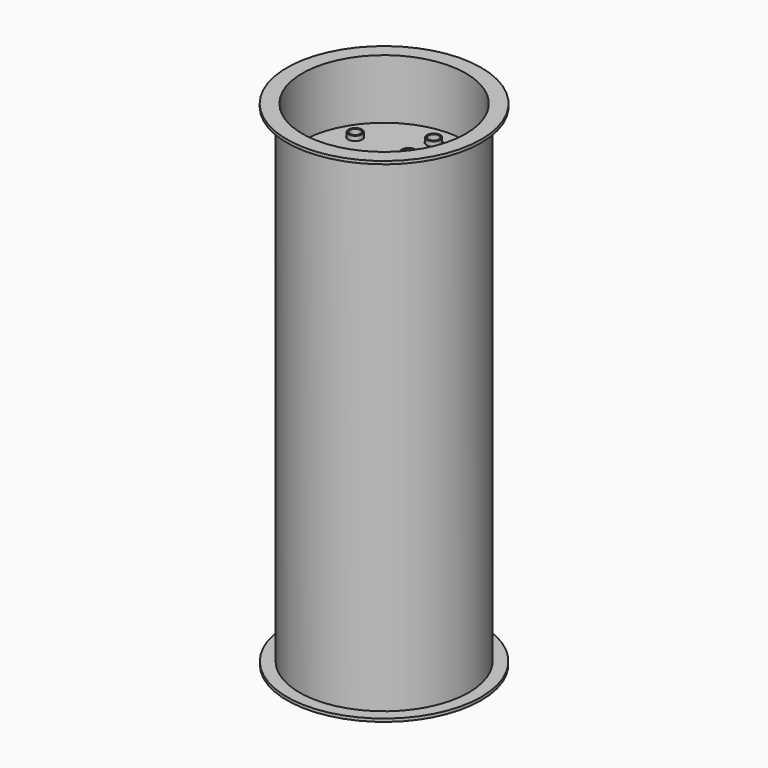
from build123d import *

# Parameters (mm, degrees)
F0_R           = 57
F0_R_2         = 55
F1_DEPTH       = 330
F3_R           = 54.5
F3_R_2         = 4.5
F3_R_3         = 4.5406250868
F4_DEPTH       = 2
F7_R           = 54.9900255747
F7_R_2         = 4.722262568
F7_R_3         = 4.8407025495
F7_R_4         = 7.5599462379
F7_R_5         = 4.9042775529
F7_R_6         = 4.7912767067
F7_R_7         = 4.7253426237
F7_R_8         = 4.6930109119
F7_R_9         = 4.737547838
F7_R_10        = 4.7706252864
F7_R_11        = 4.6617392288
F7_R_12        = 4.8204107034
F8_DEPTH       = 2
F9_R           = 65.3194518725
F9_R_2         = 57
F9_R_3         = 55
F10_DEPTH      = 2
F0_R_3         = 65.267452465
F11_DEPTH      = 2
F3_R_4         = 3.5354466149
F12_DEPTH      = 255
F12_DEPTH_BACK = 5
F3_R_5         = 3.5363153387


# Not quite as in the source:
# - a feature of the source that left no trace in its solid (it failed there, or was rolled back) is left out


with BuildPart() as f1:
    # F0 (on Top) → F1 (new body)
    with BuildSketch(Plane.XY):
        Circle(F0_R)
        Circle(F0_R_2, mode=Mode.SUBTRACT)
    extrude(amount=F1_DEPTH)

    # F9 (on face) → F10 (join)
    with BuildSketch(Plane.XY.offset(330)):
        Circle(F9_R)
        Circle(F9_R_2, mode=Mode.SUBTRACT)
        Circle(F9_R_2)
        Circle(F9_R_3, mode=Mode.SUBTRACT)
    extrude(amount=F10_DEPTH)

    # F0 (on Top) → F11 (join)
    with BuildSketch(Plane.XY):
        Circle(F0_R_3)
        Circle(F0_R, mode=Mode.SUBTRACT)
    extrude(amount=F11_DEPTH)


with BuildPart() as f4:
    # F3 (on offset) → F4 (new body)
    with BuildSketch(Plane.XY.offset(40)):
        Circle(F3_R)
        with Locations((-36.0707138286, -20.8254363388)):
            Circle(F3_R_2, mode=Mode.SUBTRACT)
        with Locations((0, -41.6508726776)):
            Circle(F3_R_2, mode=Mode.SUBTRACT)
        with Locations((0, -20.5648168921)):
            Circle(F3_R_3, mode=Mode.SUBTRACT)
        with Locations((36.0707138286, -20.8254363388)):
            Circle(F3_R_2, mode=Mode.SUBTRACT)
        with Locations((-36.0707138286, 20.8254363388)):
            Circle(F3_R_2, mode=Mode.SUBTRACT)
        with Locations((-20.5648168921, 0)):
            Circle(F3_R_3, mode=Mode.SUBTRACT)
        with Locations((20.5648168921, 0)):
            Circle(F3_R_3, mode=Mode.SUBTRACT)
        with Locations((0, 20.5648168921)):
            Circle(F3_R_3, mode=Mode.SUBTRACT)
        with Locations((36.0707138286, 20.8254363388)):
            Circle(F3_R_2, mode=Mode.SUBTRACT)
        with Locations((0, 41.6508726776)):
            Circle(F3_R_2, mode=Mode.SUBTRACT)
    extrude(amount=F4_DEPTH)


with BuildPart() as f8:
    # F7 (on offset) → F8 (new body)
    with BuildSketch(Plane.XY.offset(290)):
        Circle(F7_R)
        with Locations((-36.1077859998, -20.7854323089)):
            Circle(F7_R_2, mode=Mode.SUBTRACT)
        with Locations((0, -41.7175255716)):
            Circle(F7_R_3, mode=Mode.SUBTRACT)
        with Locations((17.5117682666, -30.032530427)):
            Circle(F7_R_4, mode=Mode.SUBTRACT)
        with Locations((0, -20.551096648)):
            Circle(F7_R_5, mode=Mode.SUBTRACT)
        with Locations((36.0051169991, -20.8520423621)):
            Circle(F7_R_6, mode=Mode.SUBTRACT)
        with Locations((-36.0934622586, 20.8296012133)):
            Circle(F7_R_7, mode=Mode.SUBTRACT)
        with Locations((-20.6031575799, 0)):
            Circle(F7_R_8, mode=Mode.SUBTRACT)
        with Locations((20.5765403807, 0)):
            Circle(F7_R_9, mode=Mode.SUBTRACT)
        with Locations((0, 20.5917563289)):
            Circle(F7_R_10, mode=Mode.SUBTRACT)
        with Locations((36.0632501543, 20.8468791097)):
            Circle(F7_R_11, mode=Mode.SUBTRACT)
        with Locations((0, 41.6552461684)):
            Circle(F7_R_12, mode=Mode.SUBTRACT)
    extrude(amount=F8_DEPTH)


with BuildPart() as f12:
    # F3 (on offset) → F12 (new body, two sides)
    with BuildSketch(Plane.XY.offset(40)) as f12_sk:
        with Locations((-36.0707138286, -20.8254363388)):
            Circle(F3_R_2)
        with Locations((-36.0707138286, -20.8254363388)):
            Circle(F3_R_4, mode=Mode.SUBTRACT)
    extrude(amount=F12_DEPTH)
    extrude(f12_sk.sketch, amount=-F12_DEPTH_BACK)


with BuildPart() as f12b:
    # F3 (on offset) → F12, piece 2 (new body, two sides)
    with BuildSketch(Plane.XY.offset(40)) as f12_2_sk:
        with Locations((-20.5648168921, 0)):
            Circle(F3_R_3)
        with Locations((-20.5648168921, 0)):
            Circle(F3_R_5, mode=Mode.SUBTRACT)
    extrude(amount=F12_DEPTH)
    extrude(f12_2_sk.sketch, amount=-F12_DEPTH_BACK)


with BuildPart() as f12c:
    # F3 (on offset) → F12, piece 3 (new body, two sides)
    with BuildSketch(Plane.XY.offset(40)) as f12_3_sk:
        with Locations((0, -41.6508726776)):
            Circle(F3_R_2)
        with Locations((0, -41.6508726776)):
            Circle(F3_R_4, mode=Mode.SUBTRACT)
    extrude(amount=F12_DEPTH)
    extrude(f12_3_sk.sketch, amount=-F12_DEPTH_BACK)


with BuildPart() as f12d:
    # F3 (on offset) → F12, piece 4 (new body, two sides)
    with BuildSketch(Plane.XY.offset(40)) as f12_4_sk:
        with Locations((36.0707138286, -20.8254363388)):
            Circle(F3_R_2)
        with Locations((36.0707138286, -20.8254363388)):
            Circle(F3_R_4, mode=Mode.SUBTRACT)
    extrude(amount=F12_DEPTH)
    extrude(f12_4_sk.sketch, amount=-F12_DEPTH_BACK)


with BuildPart() as f12e:
    # F3 (on offset) → F12, piece 5 (new body, two sides)
    with BuildSketch(Plane.XY.offset(40)) as f12_5_sk:
        with Locations((0, -20.5648168921)):
            Circle(F3_R_3)
        with Locations((0, -20.5648168921)):
            Circle(F3_R_5, mode=Mode.SUBTRACT)
    extrude(amount=F12_DEPTH)
    extrude(f12_5_sk.sketch, amount=-F12_DEPTH_BACK)


with BuildPart() as f12f:
    # F3 (on offset) → F12, piece 6 (new body, two sides)
    with BuildSketch(Plane.XY.offset(40)) as f12_6_sk:
        with Locations((36.0707138286, 20.8254363388)):
            Circle(F3_R_2)
        with Locations((36.0707138286, 20.8254363388)):
            Circle(F3_R_4, mode=Mode.SUBTRACT)
    extrude(amount=F12_DEPTH)
    extrude(f12_6_sk.sketch, amount=-F12_DEPTH_BACK)


with BuildPart() as f12g:
    # F3 (on offset) → F12, piece 7 (new body, two sides)
    with BuildSketch(Plane.XY.offset(40)) as f12_7_sk:
        with Locations((0, 41.6508726776)):
            Circle(F3_R_2)
        with Locations((0, 41.6508726776)):
            Circle(F3_R_4, mode=Mode.SUBTRACT)
    extrude(amount=F12_DEPTH)
    extrude(f12_7_sk.sketch, amount=-F12_DEPTH_BACK)


with BuildPart() as f12h:
    # F3 (on offset) → F12, piece 8 (new body, two sides)
    with BuildSketch(Plane.XY.offset(40)) as f12_8_sk:
        with Locations((0, 20.5648168921)):
            Circle(F3_R_3)
        with Locations((0, 20.5648168921)):
            Circle(F3_R_5, mode=Mode.SUBTRACT)
    extrude(amount=F12_DEPTH)
    extrude(f12_8_sk.sketch, amount=-F12_DEPTH_BACK)


with BuildPart() as f12i:
    # F3 (on offset) → F12, piece 9 (new body, two sides)
    with BuildSketch(Plane.XY.offset(40)) as f12_9_sk:
        with Locations((-36.0707138286, 20.8254363388)):
            Circle(F3_R_2)
        with Locations((-36.0707138286, 20.8254363388)):
            Circle(F3_R_4, mode=Mode.SUBTRACT)
    extrude(amount=F12_DEPTH)
    extrude(f12_9_sk.sketch, amount=-F12_DEPTH_BACK)


with BuildPart() as f12j:
    # F3 (on offset) → F12, piece 10 (new body, two sides)
    with BuildSketch(Plane.XY.offset(40)) as f12_10_sk:
        with Locations((20.5648168921, 0)):
            Circle(F3_R_3)
        with Locations((20.5648168921, 0)):
            Circle(F3_R_5, mode=Mode.SUBTRACT)
        with Locations((20.5648168921, 0)):
            Circle(F3_R_5)
    extrude(amount=F12_DEPTH)
    extrude(f12_10_sk.sketch, amount=-F12_DEPTH_BACK)


solid = Compound([f1.part, f4.part, f8.part, f12.part, f12b.part, f12c.part, f12d.part, f12e.part, f12f.part, f12g.part, f12h.part, f12i.part, f12j.part])
